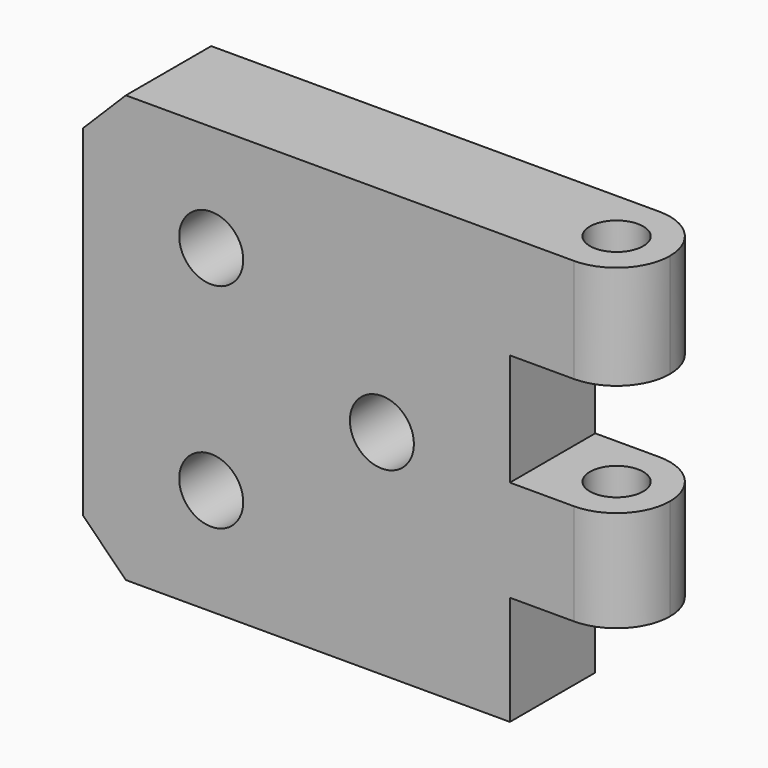
from build123d import *

# Parameters (mm, degrees)
F0_W     = 25.5
F0_H     = 20
F1_DEPTH = 5
F2_R     = 2.49999
F3_R     = 1.25
F4_DEPTH = 25
F5_W     = 9.4863112453
F5_H     = 5.25
F5_W_2   = 9.3420613807
F5_H_2   = 5.125
F6_DEPTH = 5.001
F7_R     = 1.5
F8_DEPTH = 25
F9_SIZE  = 2


# Not quite as in the source:
# - a fillet or chamfer is up to 0.001 mm smaller than in the source, because OpenCascade refuses the exact size


with BuildPart() as f1:
    # F0 (on Front) → F1 (new body)
    with BuildSketch(Plane.XZ):
        with Locations((12.75, 10)):
            Rectangle(F0_W, F0_H)
    extrude(amount=F1_DEPTH)

    # F2 (radius 2.5 in the source; OpenCascade refuses exactly that, so slightly less here)
    f2_edges = [f1.edges().sort_by_distance(p)[0] for p in [
        (25.5, -5, 10),
        (25.5, 0, 10),
    ]]
    fillet(f2_edges, radius=F2_R)

    # F3 (on face) → F4 (cut)
    with BuildSketch(Plane.XY.offset(20)):
        with Locations((23, -2.5)):
            Circle(F3_R)
    extrude(amount=-F4_DEPTH, mode=Mode.SUBTRACT)

    # F5 (on face) → F6 (cut, through all)
    with BuildSketch(Plane.XZ.offset(5)):
        with Locations((24.7431556227, 12.5)):
            Rectangle(F5_W, F5_H)
        with Locations((24.6710306904, 2.5625)):
            Rectangle(F5_W_2, F5_H_2)
    extrude(amount=-F6_DEPTH, mode=Mode.SUBTRACT)

    # F7 (on face) → F8 (cut)
    with BuildSketch(Plane.XZ.offset(5)):
        with Locations((14, 10)):
            Circle(F7_R)
        with Locations((6, 15)):
            Circle(F7_R)
        with Locations((6, 5)):
            Circle(F7_R)
    extrude(amount=-F8_DEPTH, mode=Mode.SUBTRACT)

    # F9
    f9_edges = [f1.edges().sort_by_distance(p)[0] for p in [
        (0, -2.5, 20),
        (0, -2.5, 0),
    ]]
    chamfer(f9_edges, length=F9_SIZE)


solid = f1.part
